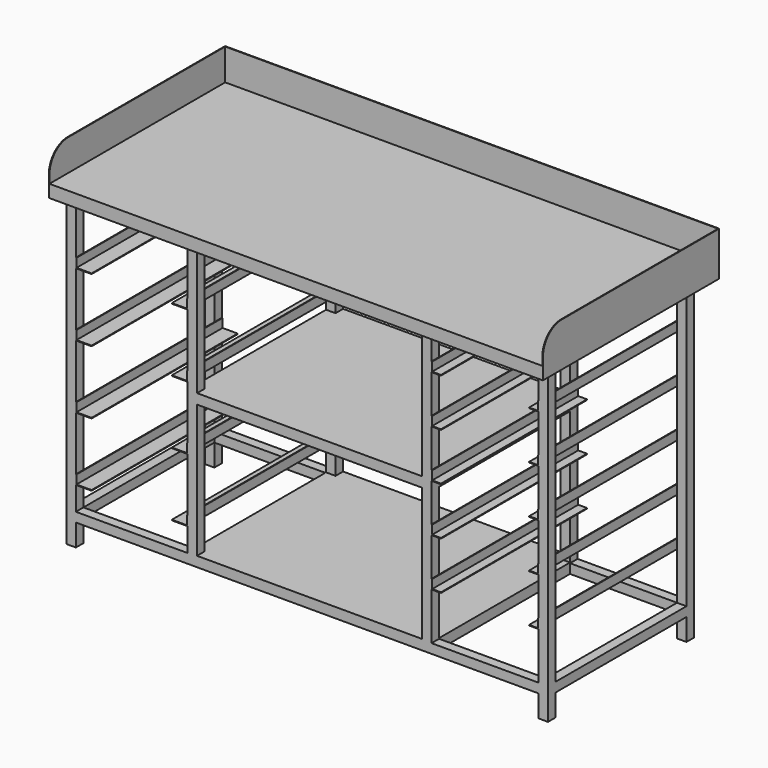
from build123d import *

# Parameters (mm, degrees)
F0_W           = 1570
F0_H           = 700
F1_DEPTH       = 40
F3_DEPTH       = 100
F4_R           = 75
F5_W           = 30
F5_H           = 30
F6_DEPTH       = 980
F7_W           = 30
F7_H           = 30
F8_DEPTH       = 735
F8_DEPTH_BACK  = 735
F9_W           = 30
F9_H           = 30
F10_DEPTH      = 275
F10_DEPTH_BACK = 245
F11_W          = 30
F11_H          = 30
F12_DEPTH      = 880
F13_W          = 30
F13_H          = 30
F14_DEPTH      = 365
F14_DEPTH_BACK = 350
F15_W          = 30
F15_H          = 30
F16_DEPTH      = 275
F16_DEPTH_BACK = 245
F18_DEPTH      = 2
F20_DEPTH      = 2
F22_DEPTH      = 580
F24_DEPTH      = 580


with BuildPart() as f1:
    # F0 (on Top) → F1 (new body)
    with BuildSketch(Plane.XY):
        Rectangle(F0_W, F0_H)
    extrude(amount=F1_DEPTH)

    # F2 (on face) → F3 (join)
    with BuildSketch(Plane.XY.offset(40)):
        Polygon((-785, 350), (-785, -350), (-783, -350), (-783, 348), (783, 348), (783, -350), (785, -350), (785, 350), align=None)
    extrude(amount=F3_DEPTH)

    # F4
    f4_edges = [f1.edges().sort_by_distance(p)[0] for p in [
        (-784, -350, 140),
        (784, -350, 140),
    ]]
    fillet(f4_edges, radius=F4_R)

    # F5 (on face) → F6 (join)
    with BuildSketch(Plane(origin=(0, 0, 0), x_dir=(1, 0, 0), z_dir=(0, 0, -1))):
        with Locations((-750, 290)):
            Rectangle(F5_W, F5_H)
        with Locations((750, 290)):
            Rectangle(F5_W, F5_H)
        with Locations((750, -260)):
            Rectangle(F5_W, F5_H)
        with Locations((-750, -260)):
            Rectangle(F5_W, F5_H)
    extrude(amount=F6_DEPTH)

    # F7 (on Right) → F8 (join, two sides)
    with BuildSketch(Plane.YZ) as f8_sk:
        with Locations((-290, -895)):
            Rectangle(F7_W, F7_H)
        with Locations((260, -895)):
            Rectangle(F7_W, F7_H)
    extrude(amount=F8_DEPTH)
    extrude(f8_sk.sketch, amount=-F8_DEPTH_BACK)

    # F9 (on Front) → F10 (join, two sides)
    with BuildSketch(Plane.XZ) as f10_sk:
        with Locations((-750, -895)):
            Rectangle(F9_W, F9_H)
        with Locations((750, -895)):
            Rectangle(F9_W, F9_H)
    extrude(amount=F10_DEPTH)
    extrude(f10_sk.sketch, amount=-F10_DEPTH_BACK)

    # F11 (on face) → F12 (join, through all)
    with BuildSketch(Plane(origin=(0, 0, 0), x_dir=(1, 0, 0), z_dir=(0, 0, -1))):
        with Locations((-365, 290)):
            Rectangle(F11_W, F11_H)
        with Locations((380, 290)):
            Rectangle(F11_W, F11_H)
        with Locations((380, -260)):
            Rectangle(F11_W, F11_H)
        with Locations((-365, -260)):
            Rectangle(F11_W, F11_H)
    extrude(amount=F12_DEPTH)

    # F13 (on Right) → F14 (join, two sides)
    with BuildSketch(Plane.YZ) as f14_sk:
        with Locations((-290, -440)):
            Rectangle(F13_W, F13_H)
        with Locations((260, -440)):
            Rectangle(F13_W, F13_H)
    extrude(amount=F14_DEPTH)
    extrude(f14_sk.sketch, amount=-F14_DEPTH_BACK)

    # F15 (on Front) → F16 (join, two sides)
    with BuildSketch(Plane.XZ) as f16_sk:
        with Locations((-365, -440)):
            Rectangle(F15_W, F15_H)
        with Locations((380, -440)):
            Rectangle(F15_W, F15_H)
        with Locations((380, -895)):
            Rectangle(F15_W, F15_H)
        with Locations((-365, -895)):
            Rectangle(F15_W, F15_H)
    extrude(amount=F16_DEPTH)
    extrude(f16_sk.sketch, amount=-F16_DEPTH_BACK)

    # F17 (on face) → F18 (join)
    with BuildSketch(Plane.XY.offset(-425)):
        Polygon((365, 245), (365, 275), (-350, 275), (-350, 245), (-380, 245), (-380, -275), (-350, -275), (-350, -305), (365, -305), (365, -275), (395, -275), (395, 245), align=None)
    extrude(amount=F18_DEPTH)

    # F19 (on face) → F20 (join)
    with BuildSketch(Plane.XY.offset(-880)):
        Polygon((365, 245), (365, 275), (-350, 275), (-350, 245), (-380, 245), (-380, -275), (-350, -275), (-350, -305), (365, -305), (365, -275), (395, -275), (395, 245), align=None)
    extrude(amount=F20_DEPTH)

    # F21 (on face) → F22 (join, through all)
    with BuildSketch(Plane.XZ.offset(305)):
        Polygon((-733, -775), (-735, -775), (-735, -805), (-685, -805), (-685, -803), (-733, -803), align=None)
        Polygon((-735, -573), (-735, -603), (-685, -603), (-685, -601), (-733, -601), (-733, -573), align=None)
        Polygon((-735, -371), (-735, -401), (-685, -401), (-685, -399), (-733, -399), (-733, -371), align=None)
        Polygon((-735, -169), (-735, -199), (-685, -199), (-685, -197), (-733, -197), (-733, -169), align=None)
        Polygon((-430, -803), (-430, -805), (-380, -805), (-380, -775), (-382, -775), (-382, -803), align=None)
        Polygon((-430, -601), (-430, -603), (-380, -603), (-380, -573), (-382, -573), (-382, -601), align=None)
        Polygon((-430, -399), (-430, -401), (-380, -401), (-380, -371), (-382, -371), (-382, -399), align=None)
        Polygon((-380, -169), (-382, -169), (-382, -197), (-430, -197), (-430, -199), (-380, -199), align=None)
    extrude(amount=-F22_DEPTH)

    # F23 (on face) → F24 (join, through all)
    with BuildSketch(Plane.XZ.offset(305)):
        Polygon((397, -700), (395, -700), (395, -730), (425, -730), (425, -728), (397, -728), align=None)
        Polygon((397, -548), (395, -548), (395, -578), (425, -578), (425, -576), (397, -576), align=None)
        Polygon((397, -396), (395, -396), (395, -426), (425, -426), (425, -424), (397, -424), align=None)
        Polygon((397, -244), (395, -244), (395, -274), (425, -274), (425, -272), (397, -272), align=None)
        Polygon((397, -92), (395, -92), (395, -122), (425, -122), (425, -120), (397, -120), align=None)
        Polygon((735, -244), (733, -244), (733, -272), (705, -272), (705, -274), (735, -274), align=None)
        Polygon((735, -92), (733, -92), (733, -120), (705, -120), (705, -122), (735, -122), align=None)
        Polygon((705, -424), (705, -426), (735, -426), (735, -396), (733, -396), (733, -424), align=None)
        Polygon((705, -730), (735, -730), (735, -700), (733, -700), (733, -728), (705, -728), align=None)
        Polygon((735, -578), (735, -548), (733, -548), (733, -576), (705, -576), (705, -578), align=None)
    extrude(amount=-F24_DEPTH)


solid = f1.part
